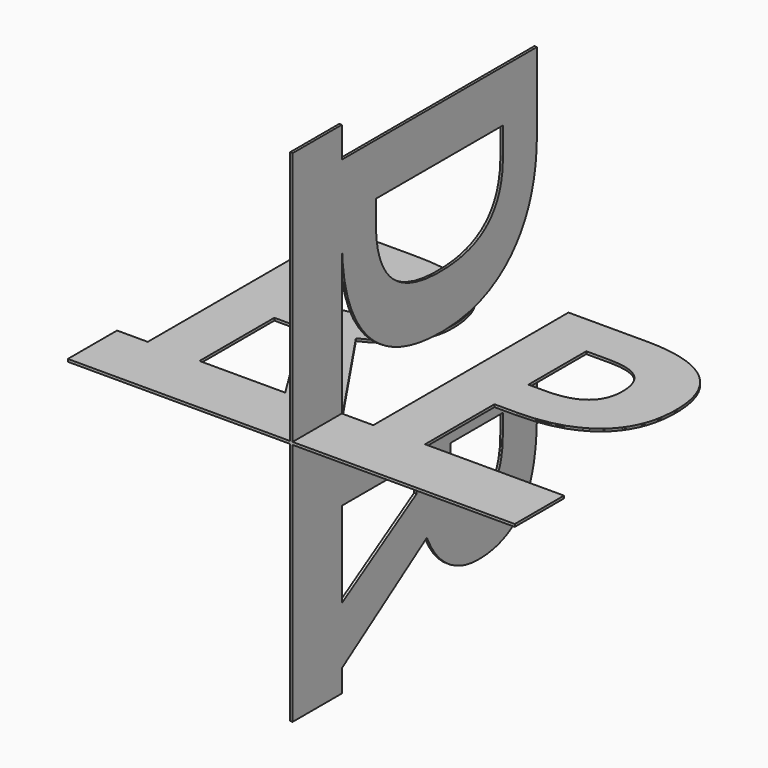
from build123d import *

# Parameters (mm, degrees)
F0_TEXT_SIZE = 423.3333333333
F1_DEPTH     = 1.5875
F2_TEXT_SIZE = 423.3333333333
F3_DEPTH     = 1.5875


# Not quite as in the source:
# - Text() gives the source's letters only with a copy of the font that has no kerning and outlines rounded to 1/6400 em; it was checked with that copy


with BuildPart() as f1:
    # F0 (on Top) → F1 (new body, symmetric)
    with BuildSketch(Plane.XY):
        Polygon((-238.81953125, 0), (-276.8533854167, 0), (-276.8533854167, -76.2), (276.8533854167, -76.2), (276.8533854167, 0), (104.7419270833, 0), (40.6466145833, 0), (2.6127604167, 0), (-68.4940104167, 0), (-174.72421875, 0), align=None)
        with Locations((-276.8533854167, 0)):
            Text('RP', F0_TEXT_SIZE, font='Open Sans', font_style=FontStyle.BOLD, text_align=(TextAlign.LEFT, TextAlign.BOTTOM))
    extrude(amount=F1_DEPTH, both=True)

    # F2 (on Right) → F3 (join, symmetric)
    with BuildSketch(Plane.YZ):
        Polygon((0, 278.4739583333), (0, 316.5078125), (-76.2, 316.5078125), (-76.2, -303.8078125), (0, -303.8078125), (0, -276.3572916667), (0, -205.2505208333), (0, -99.0203125), (0, -34.925), (0, 192.88125), align=None)
        with Locations(Location((0, 316.5078125), (0, 0, -90))):
            Text('DR', F2_TEXT_SIZE, font='Open Sans', font_style=FontStyle.BOLD, text_align=(TextAlign.LEFT, TextAlign.BOTTOM))
    extrude(amount=F3_DEPTH, both=True)


solid = f1.part
